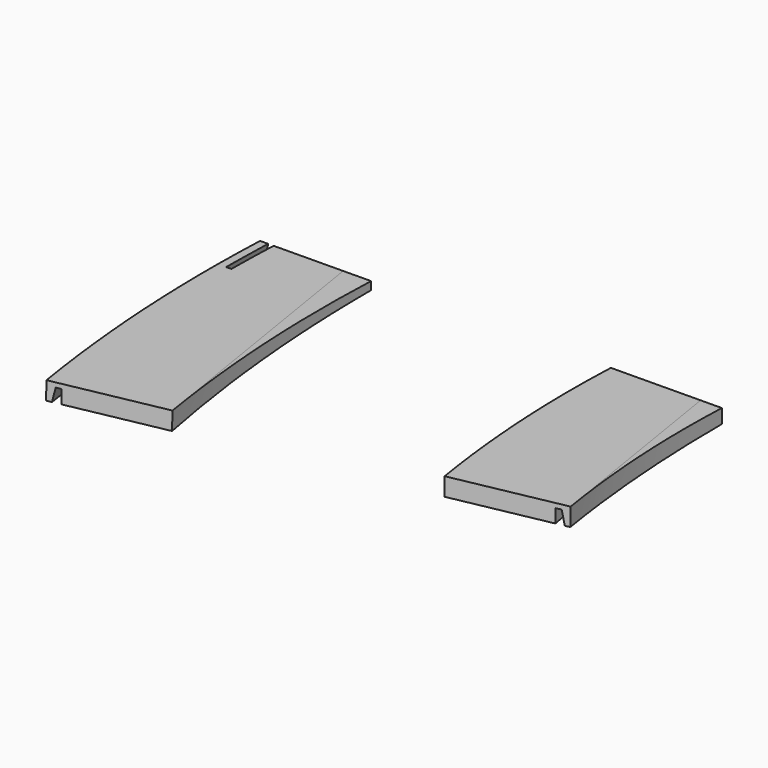
from build123d import *

# Parameters (mm, degrees)
F1_ANGLE_BACK = 11.25
F1_ANGLE      = 22.5
F2_W          = 148
F2_H          = 20.6737495929
F3_ANGLE      = 30
F5_DEPTH      = 236
F7_DEPTH      = 186.2
F8_W          = 237.9835397005
F8_H          = 111.4437803626
F9_DEPTH      = 169
F11_ANGLE     = 30
F13_ANGLE     = 2


with BuildPart() as f1:
    # F0 (on Front) → F1 (revolve)
    with BuildSketch(Plane.XZ, mode=Mode.PRIVATE) as f1_sk:
        Polygon((37.433034228, -1.662807624), (-0.066965772, -1.7883691504), (0, -21.7882570398), (37.5, -21.6626955134), align=None)
    revolve(f1_sk.sketch.rotate(Axis((525.8388087714, 0, 45.6422517605), (-0.1769446249, 0, 0.9842208084)), -F1_ANGLE_BACK), axis=Axis((525.8388087714, 0, 45.6422517605), (-0.1769446249, 0, 0.9842208084)), revolution_arc=F1_ANGLE)


with BuildPart() as f1b:
    # F0 (on Front) → F1, piece 2 (revolve)
    with BuildSketch(Plane.XZ, mode=Mode.PRIVATE) as f1_sk:
        Polygon((155.9321597647, -1.2660361285), (118.4321597647, -1.391597655), (118.4991255367, -21.3914855443), (155.9991255367, -21.2659240179), align=None)
    revolve(f1_sk.sketch.rotate(Axis((525.8388087714, 0, 45.6422517605), (-0.1769446249, 0, 0.9842208084)), -F1_ANGLE_BACK), axis=Axis((525.8388087714, 0, 45.6422517605), (-0.1769446249, 0, 0.9842208084)), revolution_arc=F1_ANGLE)


with BuildPart() as f3_tool:
    # F2 (on Front) → F3 (revolve)
    with BuildSketch(Plane.XZ):
        with Locations((78, -17.1368747965)):
            Rectangle(F2_W, F2_H)
    revolve(axis=Axis((526, 0, -14.0515491366), (0, 0, 1)), revolution_arc=F3_ANGLE)


with BuildPart() as f1_1:
    add(f1.part)

    # F3: cut by f3_tool
    add(f3_tool.part, mode=Mode.SUBTRACT)

    # F4 (on face) → F5 (cut)
    with BuildSketch(Plane(origin=(19.6894657776, -100.5725829361, 3.539800323), x_dir=(0.9813925868, 0.1918931334, -0.0067539617), z_dir=(0.1920119545, -0.9807852804, 0.0345201838))):
        Polygon((-21.0222958188, 9.4158053398), (-21.0222958188, -4.4840821492), (-9.9895421705, -4.4095212135), (-9.9949485621, -3.6095394819), (27.5044053117, -3.3561134558), (27.5098117032, -4.1560951874), (69.5515194148, -3.8719712809), (67.8833723068, 14.5498467609), align=None)
        Polygon((-9.9949485621, -3.6095394819), (-9.9895421705, -4.4095212135), (27.5098117032, -4.1560951874), (27.5044053117, -3.3561134558), align=None)
    extrude(amount=-F5_DEPTH, mode=Mode.SUBTRACT)


with BuildPart() as f1b_1:
    add(f1b.part)

    # F3: cut by f3_tool
    add(f3_tool.part, mode=Mode.SUBTRACT)

    # F6 (on face) → F7 (cut)
    with BuildSketch(Plane(origin=(19.6894657776, -100.5725829361, 3.539800323), x_dir=(0.9813925868, 0.1918931334, -0.0067539617), z_dir=(0.1920119545, -0.9807852804, 0.0345201838))):
        Polygon((100.3562242672, 19.0413011501), (98.4019598925, -3.6769958553), (108.5075416222, -3.6087008807), (108.5021352307, -2.8087191491), (146.0014891044, -2.555293123), (146.006895496, -3.3552748546), (187.190919741, -3.0769472963), (179.3207939647, 20.8833962762), align=None)
        Polygon((108.5021352307, -2.8087191491), (108.5075416222, -3.6087008807), (146.006895496, -3.3552748546), (146.0014891044, -2.555293123), align=None)
    extrude(amount=-F7_DEPTH, mode=Mode.SUBTRACT)


with BuildPart() as f9_tool:
    # F8 (on Front) → F9 (new body)
    with BuildSketch(Plane.XZ):
        with Locations((78.8098350167, -9.5459856093)):
            Rectangle(F8_W, F8_H)
    extrude(amount=-F9_DEPTH)


with BuildPart() as f1_2:
    add(f1_1.part)

    # F9: cut by f9_tool
    add(f9_tool.part, mode=Mode.SUBTRACT)


with BuildPart() as f1b_2:
    add(f1b_1.part)

    # F9: cut by f9_tool
    add(f9_tool.part, mode=Mode.SUBTRACT)


with BuildPart() as f11_tool:
    # F10 (on Front) → F11 (revolve)
    with BuildSketch(Plane.XZ):
        Polygon((1.7227589607, -8.5826770598), (0.0227684901, -8.5883691504), (0.066965772, -21.7882570398), (4.5820021559, -21.7731393102), (4.5227488708, -4.0766501403), (2.7227589607, -4.0826770598), align=None)
        Polygon((156.0660913087, -21.2659240179), (156.0218940268, -8.0660361285), (154.3219035562, -8.0717282192), (153.3219035562, -3.5717282192), (151.5219136462, -3.5777551387), (151.5811893534, -21.2809408481), align=None)
        Polygon((0.066965772, -21.7882570398), (0.0227684901, -8.5883691504), (-1.333771972, -7.7270860784), (-1.2827424282, -22.9674861319), align=None)
    revolve(axis=Axis((525.9057745435, 0, 45.6422517605), (-0.1769446249, 0, 0.9842208084)), revolution_arc=F11_ANGLE)


with BuildPart() as f1_3:
    add(f1_2.part)

    # F11: cut by f11_tool
    add(f11_tool.part, mode=Mode.SUBTRACT)

    # F12 (on Front) → F13 (revolve, cut)
    with BuildSketch(Plane.XZ):
        Polygon((2.7227589607, -2.8102906857), (2.7227589607, -4.0826770598), (4.5227488708, -4.0766501404), (4.5227488708, -2.8042637662), align=None)
    revolve(axis=Axis((525.9057745435, 0, 45.6422517605), (-0.1769446249, 0, 0.9842208084)), revolution_arc=F13_ANGLE, mode=Mode.SUBTRACT)


with BuildPart() as f1b_3:
    add(f1b_2.part)

    # F11: cut by f11_tool
    add(f11_tool.part, mode=Mode.SUBTRACT)


solid = Compound([f1_3.part, f1b_3.part])
